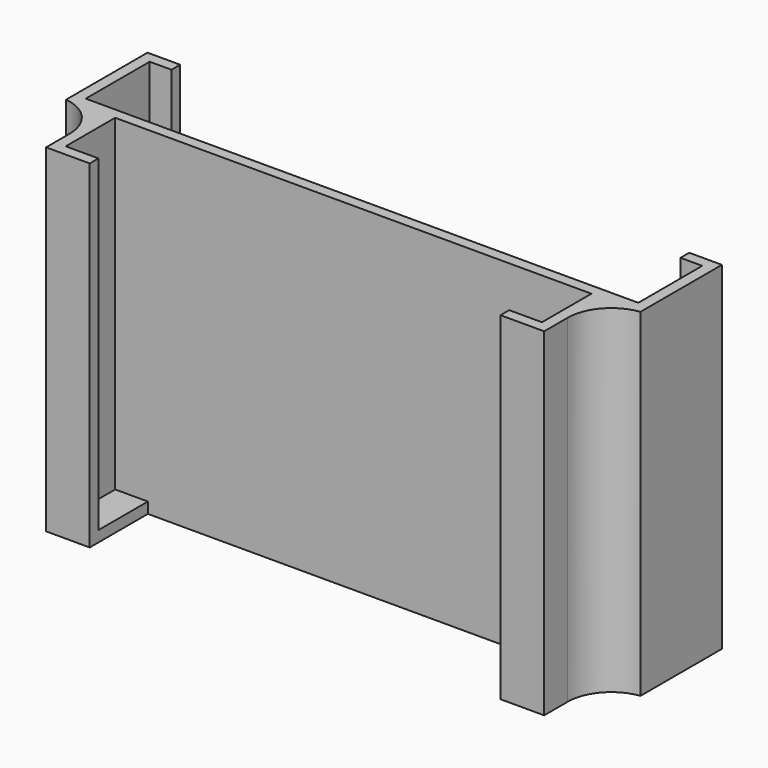
from build123d import *

# Parameters (mm, degrees)
F1_DEPTH    = 45
F2_T1_DEPTH = 45
F3_W        = 4.5
F3_H        = 8.5
F4_DEPTH    = 1.5


# Not quite as in the source:
# - a fillet or chamfer that OpenCascade refuses, or shapes differently, is made with other operations: its cross-section is extruded or revolved along the edge and cut away or added


with BuildPart() as f1:
    # F0 (on Top) → F1 (new body)
    with BuildSketch(Plane.XY):
        Polygon((38, 0), (0, 0), (-38, 0), (-38, 11), (-35, 11), (-35, 12.5), (-39.5, 12.5), (-39.5, -1.5), (-34.25, -1.5), (-32.75, -1.5), (0, -1.5), (32.75, -1.5), (34.25, -1.5), (39.5, -1.5), (39.5, 12.5), (35, 12.5), (35, 11), (38, 11), align=None)
        Polygon((-32.75, -1.5), (-34.25, -1.5), (-34.25, -11.5), (-28.25, -11.5), (-28.25, -10), (-32.75, -10), align=None)
        Polygon((34.25, -11.5), (34.25, -1.5), (32.75, -1.5), (32.75, -10), (28.25, -10), (28.25, -11.5), align=None)
    extrude(amount=F1_DEPTH)

    # F2: fillet of radius 6 on 2 edges, made by hand

    # F2_s2 → F2_t1 (join)
    with BuildSketch(Plane.XY):
        with BuildLine():
            ThreePointArc((-39.5, -1.5), (-35.75, -3.4843134833), (-34.25, -7.4529404499))
            Line((-34.25, -7.4529404499), (-34.25, -1.5))
            Line((-34.25, -1.5), (-39.5, -1.5))
        make_face()
        with BuildLine():
            ThreePointArc((34.25, -7.4529404499), (35.75, -3.4843134833), (39.5, -1.5))
            Line((39.5, -1.5), (34.25, -1.5))
            Line((34.25, -1.5), (34.25, -7.4529404499))
        make_face()
    extrude(amount=F2_T1_DEPTH)

    # F3 (on face) → F4 (join)
    with BuildSketch(Plane(origin=(0, 0, 0), x_dir=(1, 0, 0), z_dir=(0, 0, -1))):
        with BuildLine():
            Line((-32.75, 10), (-28.25, 10))
            Line((-28.25, 10), (-28.25, 11.5))
            Line((-28.25, 11.5), (-34.25, 11.5))
            Line((-34.25, 11.5), (-34.25, 7.4529404499))
            ThreePointArc((-34.25, 7.4529404499), (-35.75, 3.4843134833), (-39.5, 1.5))
            Line((-39.5, 1.5), (-39.5, -12.5))
            Line((-39.5, -12.5), (-35, -12.5))
            Line((-35, -12.5), (-35, -11))
            Line((-35, -11), (-38, -11))
            Line((-38, -11), (-38, 0))
            Line((-38, 0), (-29.5, 0))
            Line((-29.5, 0), (21.5, 0))
            Line((21.5, 0), (38, 0))
            Line((38, 0), (38, -11))
            Line((38, -11), (35, -11))
            Line((35, -11), (35, -12.5))
            Line((35, -12.5), (39.5, -12.5))
            Line((39.5, -12.5), (39.5, 1.5))
            ThreePointArc((39.5, 1.5), (35.75, 3.4843134833), (34.25, 7.4529404499))
            Line((34.25, 7.4529404499), (34.25, 11.5))
            Line((34.25, 11.5), (28.25, 11.5))
            Line((28.25, 11.5), (28.25, 10))
            Line((28.25, 10), (32.75, 10))
            Line((32.75, 10), (32.75, 1.5))
            Line((32.75, 1.5), (28.25, 1.5))
            Line((28.25, 1.5), (-28.25, 1.5))
            Line((-28.25, 1.5), (-32.75, 1.5))
            Line((-32.75, 1.5), (-32.75, 10))
        make_face()
        with Locations((-30.5, 5.75)):
            Rectangle(F3_W, F3_H)
        Polygon((-35, -11), (-35, -12.5), (-29.5, -12.5), (-29.5, 0), (-38, 0), (-38, -11), align=None)
        with Locations((30.5, 5.75)):
            Rectangle(F3_W, F3_H)
        Polygon((21.5, -12.5), (35, -12.5), (35, -11), (38, -11), (38, 0), (21.5, 0), align=None)
    extrude(amount=F4_DEPTH)


solid = f1.part
